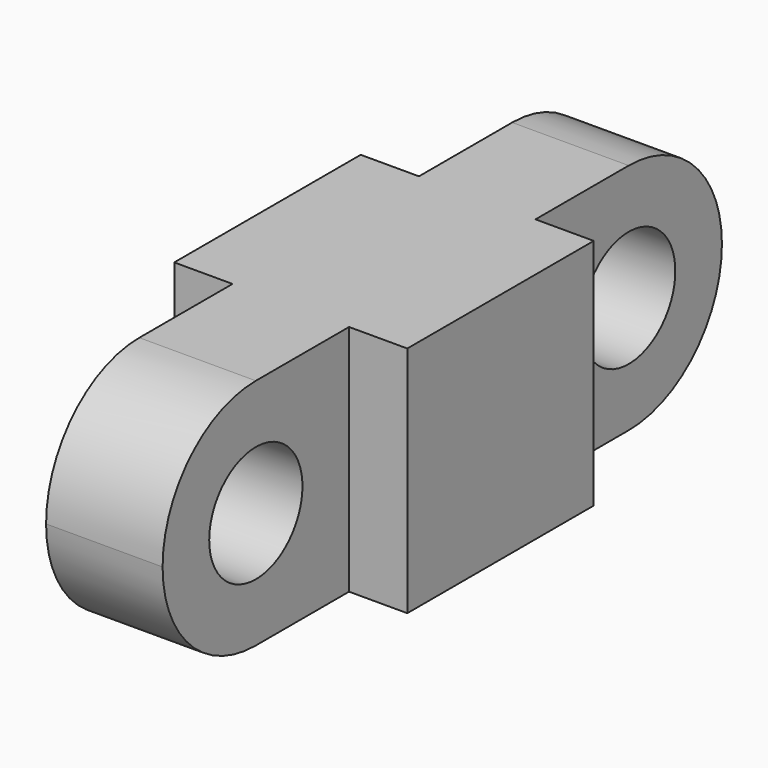
from build123d import *

# Parameters (mm, degrees)
F1_DEPTH = 40
F2_R     = 19.99999
F3_R     = 10
F4_DEPTH = 20
F5_R     = 10
F6_DEPTH = 20


# Not quite as in the source:
# - a fillet or chamfer is up to 0.001 mm smaller than in the source, because OpenCascade refuses the exact size


with BuildPart() as f1:
    # F0 (on Top) → F1 (new body)
    with BuildSketch(Plane.XY):
        Polygon((-10.9669931581, 17.3708552828), (-20.9669931581, 17.3708552828), (-20.9669931581, -22.6291447172), (-10.9669931581, -22.6291447172), (-10.9669931581, -62.6291447172), (9.0330068419, -62.6291447172), (9.0330068419, -22.6291447172), (19.0330068419, -22.6291447172), (19.0330068419, 17.3708552828), (9.0330068419, 17.3708552828), (9.0330068419, 57.3708552828), (-10.9669931581, 57.3708552828), align=None)
    extrude(amount=F1_DEPTH)

    # F2 (radius 20 in the source; OpenCascade refuses exactly that, so slightly less here)
    f2_edges = [f1.edges().sort_by_distance(p)[0] for p in [
        (-0.966993, 57.370855, 0),
        (-0.966993, 57.370855, 40),
        (-0.966993, -62.629145, 40),
        (-0.966993, -62.629145, 0),
    ]]
    fillet(f2_edges, radius=F2_R)

    # F3 (on face) → F4 (cut, through all)
    with BuildSketch(Plane(origin=(-10.9669931581, 0, 0), x_dir=(0, -1, 0), z_dir=(-1, 0, 0))):
        with Locations((-37.3708552828, 20)):
            Circle(F3_R)
    extrude(amount=-F4_DEPTH, mode=Mode.SUBTRACT)

    # F5 (on face) → F6 (cut, through all)
    with BuildSketch(Plane(origin=(-10.9669931581, 0, 0), x_dir=(0, -1, 0), z_dir=(-1, 0, 0))):
        with Locations((42.6291447172, 20)):
            Circle(F5_R)
    extrude(amount=-F6_DEPTH, mode=Mode.SUBTRACT)


solid = f1.part
